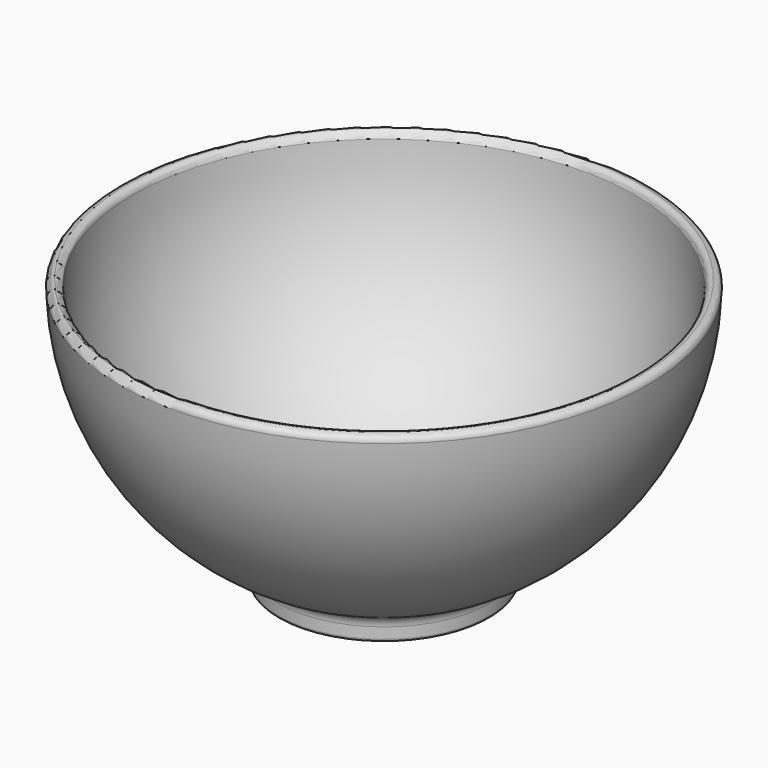
from build123d import *


# Not quite as in the source:
# - a fillet or chamfer that OpenCascade refuses, or shapes differently, is made with other operations: its cross-section is extruded or revolved along the edge and cut away or added


with BuildPart() as f1:
    # F0 (on Front) → F1 (revolve)
    with BuildSketch(Plane.XZ):
        with BuildLine():
            Line((-95.0000001118, 100), (-100, 100))
            ThreePointArc((-100, 100), (-84.5154254729, 46.5477516175), (-42.8571428571, 9.6492097095))
            ThreePointArc((-42.8571428571, 9.6492097095), (-40.7742287264, 7.8042826141), (-40, 5.1316701949))
            Line((-40, 5.1316701949), (-40, 1))
            ThreePointArc((-40, 1), (-39.7071067812, 0.2928932188), (-39, 0))
            Line((-39, 0), (-38, 0))
            ThreePointArc((-38, 0), (-37.2928932188, 0.2928932188), (-37, 1))
            Line((-37, 1), (-37, 4.1929021419))
            ThreePointArc((-37, 4.1929021419), (-36.1461786467, 5.8318879593), (-34.3137254902, 6.0714726881))
            ThreePointArc((-34.3137254902, 6.0714726881), (-17.4233646121, 1.5295660333), (0, 0))
            Line((0, 0), (0, 4.9999998882))
            ThreePointArc((0, 4.9999998882), (-67.1751442917, 32.8248557083), (-95.0000001118, 100))
        make_face()
    revolve(axis=Axis((0, 0, 2.4999999441), (0, 0, -1)))

    # F2: fillet of radius 2.5 on 2 edges, made by hand

    # F2_s1 → F2_t2 (revolve, cut)
    with BuildSketch(Plane.XZ):
        with BuildLine():
            ThreePointArc((-97.4679434481, 100), (-99.2582306332, 99.2449561011), (-99.9671214852, 97.4358974359))
            ThreePointArc((-99.9671214852, 97.4358974359), (-99.9917800335, 98.7178433251), (-100, 100))
            Line((-100, 100), (-97.4679434481, 100))
        make_face()
    revolve(axis=Axis((0, 0, 100), (0, 0, -1)), mode=Mode.SUBTRACT)

    # F2_s3 → F2_t4 (revolve, cut)
    with BuildSketch(Plane.XZ):
        with BuildLine():
            ThreePointArc((-94.9687655228, 97.564102564), (-95.7229874587, 99.2902871851), (-97.4679435599, 100))
            Line((-97.4679435599, 100), (-95.0000001118, 100))
            ThreePointArc((-95.0000001118, 100), (-94.9921911436, 98.7819511588), (-94.9687655228, 97.564102564))
        make_face()
    revolve(axis=Axis((0, 0, 100), (0, 0, -1)), mode=Mode.SUBTRACT)


solid = f1.part
